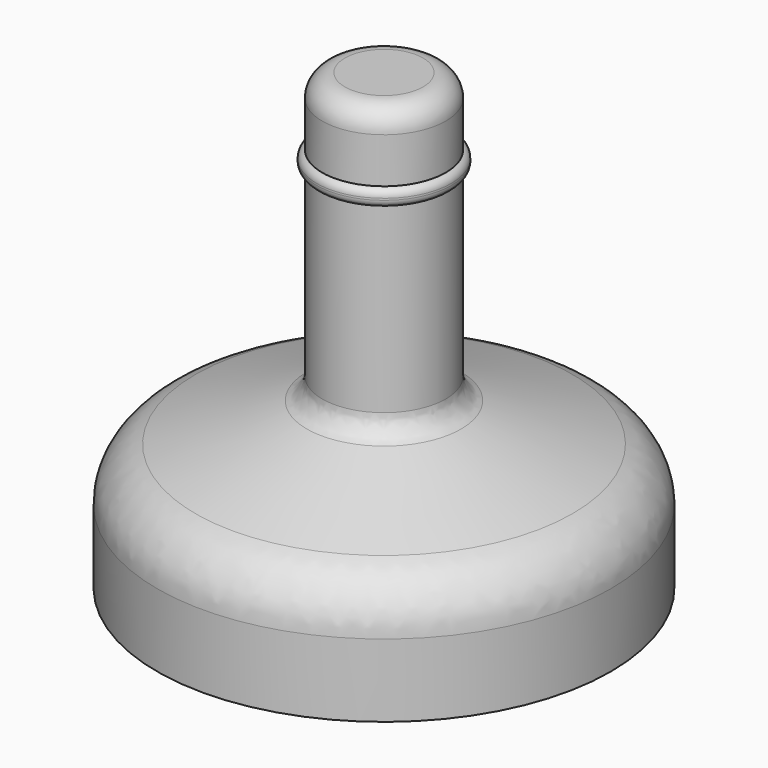
from build123d import *

# Parameters (mm, degrees)
F0_W = 0.5
F0_H = 1.5
F2_R = 2
F3_R = 5


# Not quite as in the source:
# - a fillet or chamfer that OpenCascade refuses, or shapes differently, is made with other operations: its cross-section is extruded or revolved along the edge and cut away or added


with BuildPart() as f1:
    # F0 (on Front) → F1 (revolve)
    with BuildSketch(Plane.XZ):
        Polygon((0, 40), (0, 0), (20, 0), (20, 10), (5.45, 15), (5.45, 32.5), (5.45, 34), (5.45, 40), align=None)
        with Locations((5.7, 33.25)):
            Rectangle(F0_W, F0_H)
    revolve(axis=Axis((0, 0, 20), (0, 0, 1)))

    # F2
    f2_edges = [f1.edges().sort_by_distance(p)[0] for p in [
        (-5.45, 0, 40),
        (-5.45, 0, 15),
    ]]
    fillet(f2_edges, radius=F2_R)

    # F3
    f3_edges = [f1.edges().sort_by_distance(p)[0] for p in [
        (-20, 0, 10),
    ]]
    fillet(f3_edges, radius=F3_R)

    # F4: fillet of radius 0.7 on 3 edges, made by hand

    # F4_s1 → F4_t2 (revolve, cut)
    with BuildSketch(Plane.XZ):
        with BuildLine():
            ThreePointArc((5.45, 32.5), (5.811248608, 32.75249038), (5.95, 33.1708203932))
            Line((5.95, 33.1708203932), (5.95, 32.5))
            Line((5.95, 32.5), (5.45, 32.5))
        make_face()
    revolve(axis=Axis((0, 0, 32.5), (0, 0, 1)), mode=Mode.SUBTRACT)

    # F4_s3 → F4_t4 (revolve, cut)
    with BuildSketch(Plane.XZ):
        with BuildLine():
            ThreePointArc((5.95, 33.3291796068), (5.811248608, 33.74750962), (5.45, 34))
            Line((5.45, 34), (5.95, 34))
            Line((5.95, 34), (5.95, 33.3291796068))
        make_face()
    revolve(axis=Axis((0, 0, 34), (0, 0, 1)), mode=Mode.SUBTRACT)


solid = f1.part
